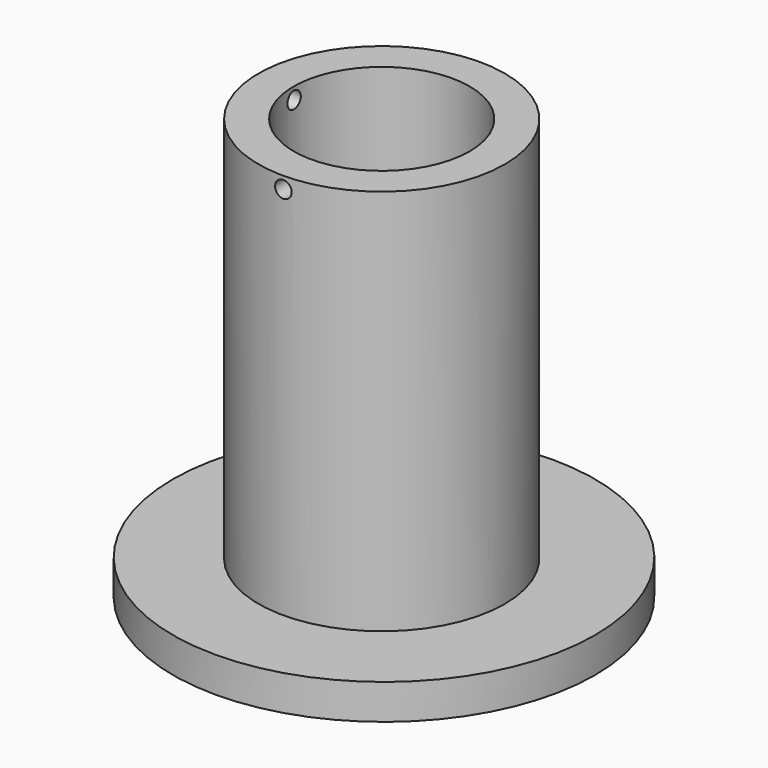
from build123d import *

# Parameters (mm, degrees)
F0_R            = 22.225
F0_R_2          = 15.875
F1_DEPTH        = 76.2
F2_R            = 1.5
F3_DEPTH        = 25
F3_COPIES_COUNT = 2
F3_COPIES_ANGLE = 90
F4_R            = 38.1
F4_R_2          = 22.225
F5_DEPTH        = 6.35


# Not quite as in the source:
# - a pattern or mirror of a feature is missing from the dataset's text; its kind, count and spacing are read off the source's solid


with BuildPart() as f1:
    # F0 (on Top) → F1 (new body)
    with BuildSketch(Plane.XY):
        Circle(F0_R)
        Circle(F0_R_2, mode=Mode.SUBTRACT)
    extrude(amount=F1_DEPTH)

    # F2 (on Right) → F3 (cut)
    with BuildSketch(Plane.YZ):
        with Locations((0, 74.041)):
            Circle(F2_R)
    f3 = extrude(amount=-F3_DEPTH, mode=Mode.SUBTRACT)

    # F3_copies: F3 ×2 about axis
    f3_copies_axis = Axis((0, 0, 0), (0, 0, 1))
    for i in range(1, F3_COPIES_COUNT):
        add(f3.rotate(f3_copies_axis, i * F3_COPIES_ANGLE / (F3_COPIES_COUNT - 1)), mode=Mode.SUBTRACT)

    # F4 (on face) → F5 (join)
    with BuildSketch(Plane(origin=(0, 0, 0), x_dir=(1, 0, 0), z_dir=(0, 0, -1))):
        with Locations((0, -0.5167627824)):
            Circle(F4_R)
        Circle(F4_R_2, mode=Mode.SUBTRACT)
    extrude(amount=-F5_DEPTH)


solid = f1.part
